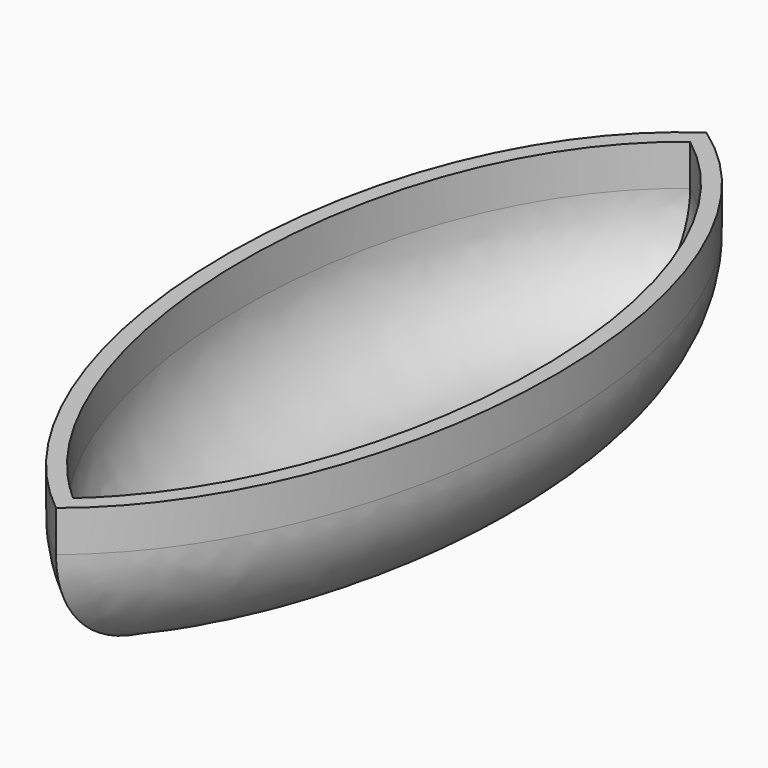
from build123d import *

# Parameters (mm, degrees)
F1_DEPTH = 25.4
F2_R     = 19.05
F3_T     = 2.54


# Not quite as in the source:
# - a shell that OpenCascade refuses in one call is made with other operations: the cavity is built on its own and cut out


with BuildPart() as f1:
    # F0 (on Top) → F1 (new body)
    with BuildSketch(Plane.XY):
        with BuildLine():
            add(Edge.make_bspline(
                [(0, 61.2068687557), (34.7973253535, 37.2046761593), (32.9233254877, -38.4026963533), (0, -64.7510275931)],
                knots=[0, 0, 0, 0, 125.9578963488, 125.9578963488, 125.9578963488, 125.9578963488], degree=3))
            add(Edge.make_bspline(
                [(0, 61.2068687557), (-34.7973253535, 37.2046761593), (-32.9233254877, -38.4026963533), (0, -64.7510275931)],
                knots=[0, 0, 0, 0, 125.9578963488, 125.9578963488, 125.9578963488, 125.9578963488], degree=3))
        make_face()
    extrude(amount=F1_DEPTH)

    # F2
    f2_edges = [f1.edges().sort_by_distance(p)[0] for p in [
        (25.388279, -1.477706, 0),
        (-25.388279, -1.477706, 0),
    ]]
    fillet(f2_edges, radius=F2_R)

    # F3: shell of thickness 2.54, made by hand


with BuildPart() as f3_core1:
    # F3_t2: copy of F1
    add(f1.part)

    # the walls: a layer under each face that stays
    f3_faces = [f3_core1.faces().sort_by_distance(p)[0] for p in [
        (25.3952440654, -0.8922774275, 22.2249999997),
        (-25.3952440654, -0.8922774275, 22.2249999997),
        (19.8158692116, -0.8404055925, 5.5796158184),
        (-19.8158692116, -0.8404055925, 5.5796158184),
        (0, -0.567489107, 0),
    ]]
    thicken(f3_faces, amount=-F3_T, mode=Mode.SUBTRACT)


with BuildPart() as f1_1:
    add(f1.part)

    # what is left inside the walls is the cavity
    f3_cavity = [f3_core1.part.solids().sort_by_distance(p)[0] for p in [
        (0, -21.599264, 25.3746),
    ]]
    add(f3_cavity, mode=Mode.SUBTRACT)


solid = f1_1.part
